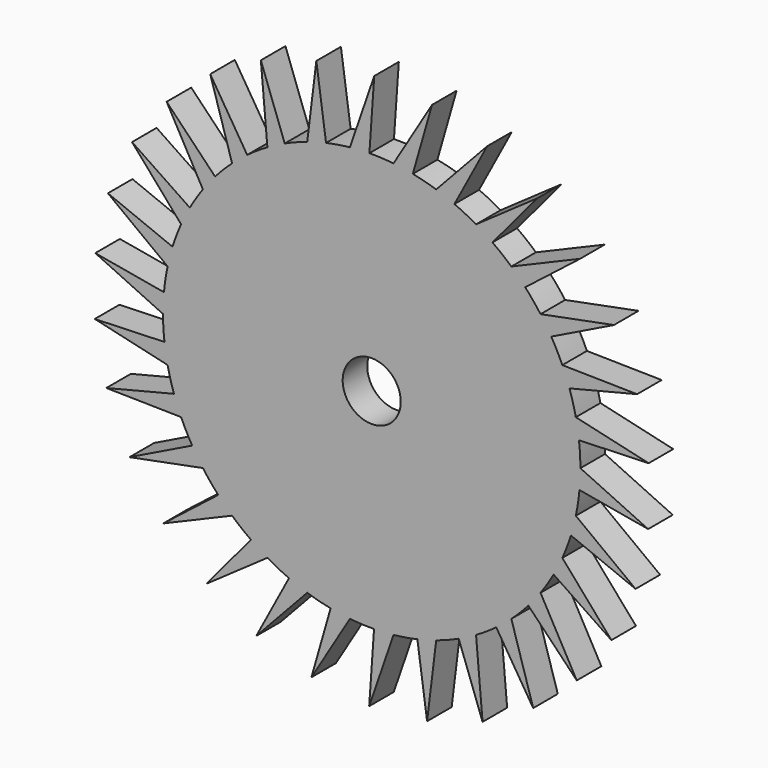
from build123d import *

# Parameters (mm, degrees)
F0_R            = 1.5
F1_DEPTH        = 1.5875
F1_COPIES_COUNT = 30
F2_DEPTH        = 1.5875


# Not quite as in the source:
# - a length typed as a fraction of an inch, garbled in the dataset ("3 / 203.2 mm" for 3/8 in), is restored
# - a pattern or mirror of a feature is missing from the dataset's text; its kind, count and spacing are read off the source's solid


with BuildPart() as f1:
    # F0 (on Front) → F1 (new body)
    with BuildSketch(Plane.XZ):
        with BuildLine():
            ThreePointArc((-10.7832175985, 0), (0, -10.7832175985), (10.7832175985, 0))
            ThreePointArc((10.7832175985, 0), (0.5040652179, 10.7714298045), (-10.7360921943, 1.0070283867))
            ThreePointArc((-10.7360921943, 1.0070283867), (-10.7714298045, 0.5040652179), (-10.7832175985, 0))
        make_face()
        Circle(F0_R, mode=Mode.SUBTRACT)
        with BuildLine():
            ThreePointArc((-10.7832175985, 0), (-10.7714298045, 0.5040652179), (-10.7360921943, 1.0070283867))
            Line((-10.7360921943, 1.0070283867), (-14.2846159535, 1.6327288672))
            Line((-14.2846159535, 1.6327288672), (-10.7832175985, 0))
        make_face()
    extrude(amount=F1_DEPTH)

    # F1_copies: F1 ×30 about axis
    f1_copies_axis = Axis((0, 0, 0), (0, 1, 0))


with BuildPart() as f1_1:
    add(f1.part)
    for i in range(1, F1_COPIES_COUNT):
        add(f1.part.rotate(f1_copies_axis, i * 360 / F1_COPIES_COUNT))

    # F0 (on Front) → F2 (join)
    with BuildSketch(Plane.XZ):
        with BuildLine():
            ThreePointArc((-10.7832175985, 0), (0, -10.7832175985), (10.7832175985, 0))
            ThreePointArc((10.7832175985, 0), (0.5040652179, 10.7714298045), (-10.7360921943, 1.0070283867))
            ThreePointArc((-10.7360921943, 1.0070283867), (-10.7714298045, 0.5040652179), (-10.7832175985, 0))
        make_face()
        Circle(F0_R, mode=Mode.SUBTRACT)
        with BuildLine():
            ThreePointArc((-10.7832175985, 0), (-10.7714298045, 0.5040652179), (-10.7360921943, 1.0070283867))
            Line((-10.7360921943, 1.0070283867), (-14.2846159535, 1.6327288672))
            Line((-14.2846159535, 1.6327288672), (-10.7832175985, 0))
        make_face()
    extrude(amount=F2_DEPTH)


solid = f1_1.part
